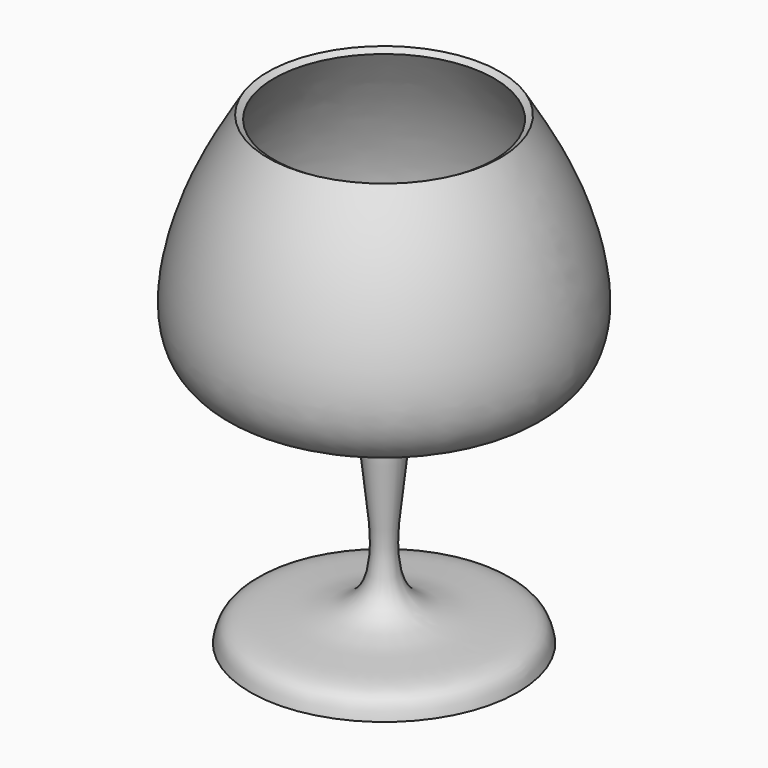
from build123d import *


# Not quite as in the source:
# - ends of sketch curves that miss each other by under 0.0002 mm in the source are joined
# - the dataset's text gives a spline's control points without its knots; the knots are read off the source's solid


with BuildPart() as f1:
    # F0 (on Front) → F1 (revolve)
    with BuildSketch(Plane.XZ):
        with BuildLine():
            Line((0, 0), (23.3897306025, 0))
            add(Edge.make_bspline(
                [(23.3897306025, 0), (23.0811798378, 1.4225812529), (22.1483800237, 5.7232788373), (-4.0570977705, 1.5105508976), (5.7598610272, 32.5010243601), (-0.9454321257, 40.0805419146), (33.9920769176, 36.5900877138), (29.9851488557, 65.348679349), (23.5089253895, 76.0477686392), (20.340019837, 81.2829807401)],
                knots=[0, 0, 0, 0, 0.0754198046, 0.2280064994, 0.4105345247, 0.4917705589, 0.6705421429, 0.838791722, 1, 1, 1, 1], degree=3))
            Line((20.340019837, 81.2829807401), (19.2535555125, 80.6253373124))
            add(Edge.make_bspline(
                [(1.4687033423, 37.9807189459), (1.4917544156, 38.0223281839), (1.58238803, 38.1741146427), (1.8513600454, 38.5195676029), (2.3518478608, 38.9007735045), (2.9857016516, 39.1820426358), (3.6659397339, 39.3839249896), (4.4175915194, 39.5398011877), (5.2465714411, 39.6656456284), (6.4546814047, 39.8052480611), (8.1468147671, 39.943506941), (10.4094502803, 40.0930615542), (12.8307393668, 40.2632395293), (15.3321339566, 40.4898116951), (17.8315460182, 40.8073186483), (20.2438677318, 41.2484287549), (22.4812150553, 41.8422920864), (24.1232066058, 42.4822959216), (25.2606781167, 43.0859163853), (26.0126529085, 43.5812118276), (26.6732225892, 44.1280379986), (27.4502369596, 44.9280821369), (28.2405364896, 46.0583886916), (28.9342379496, 47.6217661888), (29.3886791208, 49.376449929), (29.6941949541, 51.9303067104), (29.5553060802, 55.4289549611), (28.8831071859, 59.0651252809), (28.1393600861, 61.9009651867), (27.2997558906, 64.6347945785), (26.1302000679, 67.7900849021), (24.5644522425, 71.2592564884), (22.8733235274, 74.4963036898), (21.0915466535, 77.5887736478), (19.8678434372, 79.6104987432), (19.2535555125, 80.6253373124)],
                knots=[0.4790230117, 0.4790230117, 0.4790230117, 0.4790230117, 0.48046875, 0.484375, 0.4921875, 0.5, 0.5078125, 0.515625, 0.5234375, 0.53125, 0.546875, 0.5625, 0.578125, 0.59375, 0.609375, 0.625, 0.640625, 0.65625, 0.6640625, 0.671875, 0.6796875, 0.6875, 0.703125, 0.71875, 0.734375, 0.75, 0.78125, 0.8125, 0.828125, 0.84375, 0.875, 0.90625, 0.9375, 0.96875, 1, 1, 1, 1], degree=3))
            Line((1.4687033423, 37.9807189459), (0, 37.9807466314))
            Line((0, 37.9807466314), (0, 0))
        make_face()
    revolve(axis=Axis((0, 0, 18.9903733157), (0, 0, -1)))


solid = f1.part
